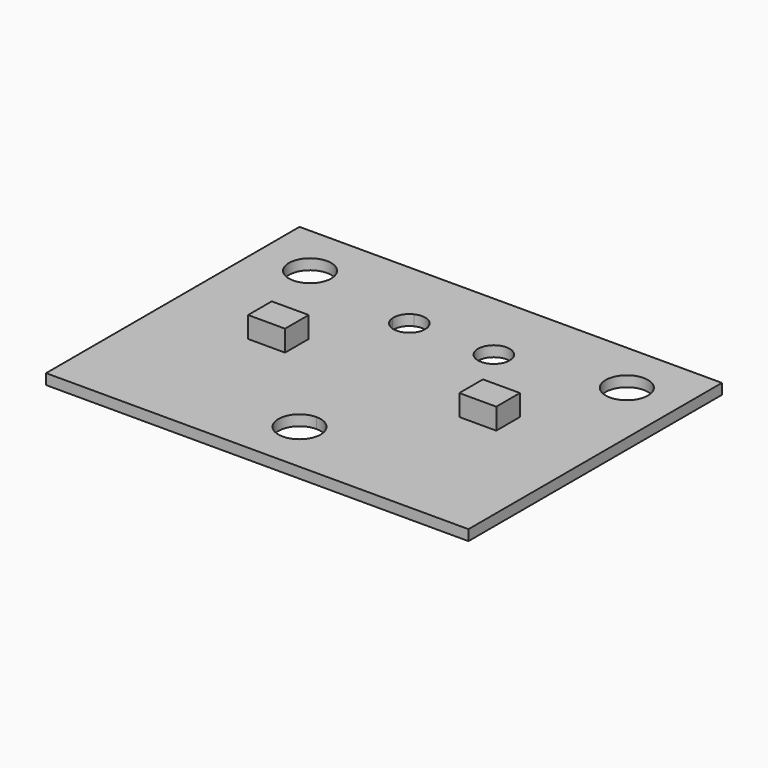
from build123d import *

# Parameters (mm, degrees)
F0_R     = 2
F1_DEPTH = 1
F2_DEPTH = 3


with BuildPart() as f1:
    # F0 (on Top) → F1 (new body)
    with BuildSketch(Plane.XY):
        with BuildLine():
            Line((0, 30), (0, 0))
            Line((0, 0), (20, 0))
            Line((20, 0), (20, 0.5))
            ThreePointArc((20, 0.5), (15.5, 5), (20, 9.5))
            Line((20, 9.5), (5, 9.5))
            Line((5, 9.5), (5, 20.5))
            Line((5, 20.5), (13.1542079159, 20.5))
            Line((13.1542079159, 20.5), (14.5067032721, 22.8583494358))
            ThreePointArc((14.5067032721, 22.8583494358), (14.6987936477, 23.7462318867), (15.3681283209, 24.3604183846))
            Line((15.3681283209, 24.3604183846), (18.6023852252, 30))
            Line((18.6023852252, 30), (0, 30))
        make_face()
        with BuildLine():
            ThreePointArc((9.5, 25), (8.1819805153, 21.8180194847), (5, 20.5))
            ThreePointArc((5, 20.5), (1.8180194847, 28.1819805153), (9.5, 25))
        make_face(mode=Mode.SUBTRACT)
        Polygon((5, 9.5), (20, 9.5), (20, 20.5), (13.1542079159, 20.5), (5, 20.5), align=None)
        Polygon((8.25, 16.4), (10.8028892877, 16.4), (11.75, 16.4), (11.75, 13.6), (8.25, 13.6), align=None, mode=Mode.SUBTRACT)
        Polygon((27.5459935813, 9.5), (29.8604090717, 0), (40, 0), (40, 9.5), (35, 9.5), align=None)
        Polygon((24.866144066, 20.5), (27.5459935813, 9.5), (35, 9.5), (35, 20.5), (28.6657820621, 20.5), align=None)
        Polygon((28.25, 16.4), (29.6603808885, 16.4), (31.75, 16.4), (31.75, 13.6), (28.25, 13.6), align=None, mode=Mode.SUBTRACT)
        Polygon((26.3612238059, 30), (20, 30), (20, 20.5), (24.866144066, 20.5), (28.6657820621, 20.5), align=None)
        with BuildLine():
            ThreePointArc((25.5, 23), (25.2528295373, 22.1751253729), (24.5927757995, 21.6220969368))
            ThreePointArc((24.5927757995, 21.6220969368), (22.7471704627, 23.8248746271), (25.5, 23))
        make_face(mode=Mode.SUBTRACT)
        Polygon((20, 20.5), (20, 9.5), (27.5459935813, 9.5), (24.866144066, 20.5), align=None)
        with BuildLine():
            ThreePointArc((9.5, 25), (1.8180194847, 28.1819805153), (5, 20.5))
            ThreePointArc((5, 20.5), (8.1819805153, 21.8180194847), (9.5, 25))
        make_face()
        with Locations((5, 25)):
            Circle(F0_R, mode=Mode.SUBTRACT)
        with BuildLine():
            ThreePointArc((39.5, 25), (31.8180194847, 28.1819805153), (35, 20.5))
            ThreePointArc((35, 20.5), (37.8235020538, 21.4960256633), (39.3971016605, 24.0431839323))
            ThreePointArc((39.3971016605, 24.0431839323), (39.4742014635, 24.5188334343), (39.5, 25))
        make_face()
        with Locations((35, 25)):
            Circle(F0_R, mode=Mode.SUBTRACT)
        with BuildLine():
            Line((35, 9.5), (40, 9.5))
            Line((40, 9.5), (40, 23.9542004244))
            Line((40, 23.9542004244), (39.3971016605, 24.0431839323))
            ThreePointArc((39.3971016605, 24.0431839323), (37.8235020538, 21.4960256633), (35, 20.5))
            Line((35, 20.5), (35, 9.5))
        make_face()
        with BuildLine():
            Line((40, 30), (26.3612238059, 30))
            Line((26.3612238059, 30), (28.6657820621, 20.5))
            Line((28.6657820621, 20.5), (35, 20.5))
            ThreePointArc((35, 20.5), (31.8180194847, 28.1819805153), (39.5, 25))
            ThreePointArc((39.5, 25), (39.4742014635, 24.5188334343), (39.3971016605, 24.0431839323))
            Line((39.3971016605, 24.0431839323), (40, 23.9542004244))
            Line((40, 23.9542004244), (40, 30))
        make_face()
        with BuildLine():
            Line((23.4659308964, 2.1299263039), (26.0225208067, 0))
            Line((26.0225208067, 0), (29.8604090717, 0))
            Line((29.8604090717, 0), (27.5459935813, 9.5))
            Line((27.5459935813, 9.5), (20, 9.5))
            ThreePointArc((20, 9.5), (23.1819805153, 8.1819805153), (24.5, 5))
            ThreePointArc((24.5, 5), (24.2335971132, 3.4746621741), (23.4659308964, 2.1299263039))
        make_face()
        with BuildLine():
            Line((20, 30), (18.6023852252, 30))
            Line((18.6023852252, 30), (15.3681283209, 24.3604183846))
            ThreePointArc((15.3681283209, 24.3604183846), (16.806905348, 24.2644776627), (17.5, 23))
            ThreePointArc((17.5, 23), (16.0709045418, 21.5016767552), (14.5067032721, 22.8583494358))
            Line((14.5067032721, 22.8583494358), (13.1542079159, 20.5))
            Line((13.1542079159, 20.5), (20, 20.5))
            Line((20, 20.5), (20, 30))
        make_face()
        with BuildLine():
            ThreePointArc((20, 9.5), (15.5, 5), (20, 0.5))
            Line((20, 0.5), (20, 3))
            ThreePointArc((20, 3), (18, 5), (20, 7))
            Line((20, 7), (20, 9.5))
        make_face()
        with BuildLine():
            Line((21.5451496956, 3.7301526004), (23.4659308964, 2.1299263039))
            ThreePointArc((23.4659308964, 2.1299263039), (24.2335971132, 3.4746621741), (24.5, 5))
            ThreePointArc((24.5, 5), (23.1819805153, 8.1819805153), (20, 9.5))
            Line((20, 9.5), (20, 7))
            ThreePointArc((20, 7), (21.4142135624, 6.4142135624), (22, 5))
            ThreePointArc((22, 5), (21.882856791, 4.3255740927), (21.5451496956, 3.7301526004))
        make_face()
        Polygon((11.75, 16.4), (10.8028892877, 16.4), (8.25, 16.4), (8.25, 13.6), (11.75, 13.6), align=None)
        Polygon((31.75, 16.4), (29.6603808885, 16.4), (28.25, 16.4), (28.25, 13.6), (31.75, 13.6), align=None)
        with BuildLine():
            Line((20, 3), (20, 0.5))
            ThreePointArc((20, 0.5), (21.9150285073, 0.9278180522), (23.4659308964, 2.1299263039))
            Line((23.4659308964, 2.1299263039), (21.5451496956, 3.7301526004))
            ThreePointArc((21.5451496956, 3.7301526004), (20.8544896725, 3.1917280626), (20, 3))
        make_face()
        with BuildLine():
            Line((20, 0.5), (20, 0))
            Line((20, 0), (26.0225208067, 0))
            Line((26.0225208067, 0), (23.4659308964, 2.1299263039))
            ThreePointArc((23.4659308964, 2.1299263039), (21.9150285073, 0.9278180522), (20, 0.5))
        make_face()
    extrude(amount=F1_DEPTH)


with BuildPart() as f2:
    # F0 (on Top) → F2 (new body)
    with BuildSketch(Plane.XY):
        Polygon((31.75, 16.4), (29.6603808885, 16.4), (28.25, 16.4), (28.25, 13.6), (31.75, 13.6), align=None)
    extrude(amount=F2_DEPTH)


with BuildPart() as f2b:
    # F0 (on Top) → F2, piece 2 (new body)
    with BuildSketch(Plane.XY):
        Polygon((11.75, 16.4), (10.8028892877, 16.4), (8.25, 16.4), (8.25, 13.6), (11.75, 13.6), align=None)
    extrude(amount=F2_DEPTH)


solid = Compound([f1.part, f2.part, f2b.part])
